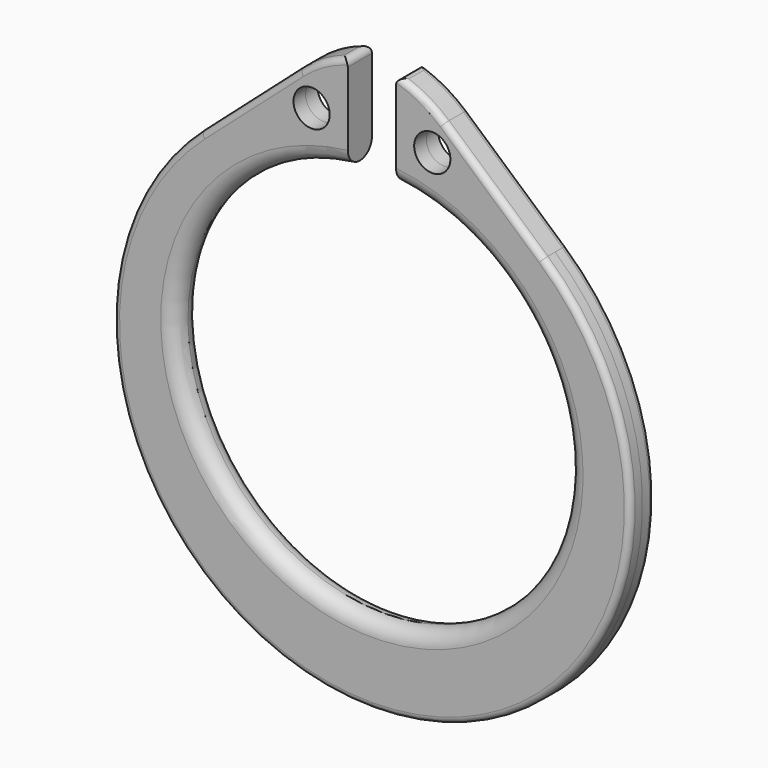
from build123d import *

# Parameters (mm, degrees)
F0_R     = 1.5
F1_DEPTH = 1.25
F2_R     = 1.24999
F3_R     = 0.5


# Not quite as in the source:
# - a fillet or chamfer is up to 0.001 mm smaller than in the source, because OpenCascade refuses the exact size


with BuildPart() as f1:
    # F0 (on Front) → F1 (new body, symmetric)
    with BuildSketch(Plane.XZ):
        with BuildLine():
            ThreePointArc((2, 16.1264534229), (0, -16.25), (-2, 16.1264534229))
            Line((-2, 16.1264534229), (-2, 24.1264534229))
            ThreePointArc((-2, 24.1264534229), (-4.1221023219, 23.2646436342), (-5.9979579511, 21.9504138084))
            Line((-5.9979579511, 21.9504138084), (-14.1837464065, 14.7155008072))
            ThreePointArc((-14.1837464065, 14.7155008072), (-20.0302422156, -8.9154770598), (0, -22.75))
            ThreePointArc((0, -22.75), (20.0302422156, -8.9154770598), (14.1837464065, 14.7155008072))
            Line((14.1837464065, 14.7155008072), (5.9979579511, 21.9504138084))
            ThreePointArc((5.9979579511, 21.9504138084), (4.1221023219, 23.2646436342), (2, 24.1264534229))
            Line((2, 24.1264534229), (2, 16.1264534229))
        make_face()
        with Locations((-5, 19.4933966718)):
            Circle(F0_R, mode=Mode.SUBTRACT)
        with Locations((5, 19.4933966718)):
            Circle(F0_R, mode=Mode.SUBTRACT)
    extrude(amount=F1_DEPTH, both=True)

    # F2 (radius 1.25 in the source; OpenCascade refuses exactly that, so slightly less here)
    f2_edges = [f1.edges().sort_by_distance(p)[0] for p in [
        (0, -1.25, -16.25),
        (0, 1.25, -16.25),
    ]]
    fillet(f2_edges, radius=F2_R)

    # F3
    f3_edges = [f1.edges().sort_by_distance(p)[0] for p in [
        (-20.030242, -1.25, -8.915477),
        (20.030242, -1.25, -8.915477),
        (-20.030242, 1.25, -8.915477),
        (20.030242, 1.25, -8.915477),
        (10.090852, 1.25, 18.332957),
        (10.090852, -1.25, 18.332957),
        (4.122102, -1.25, 23.264644),
        (4.122102, 1.25, 23.264644),
        (2, 0.625, 24.126453),
        (2, -0.625, 24.126453),
        (-10.090852, -1.25, 18.332957),
        (-10.090852, 1.25, 18.332957),
        (-4.122102, -1.25, 23.264644),
        (-4.122102, 1.25, 23.264644),
        (-2, 0.625, 24.126453),
        (-2, -0.625, 24.126453),
    ]]
    fillet(f3_edges, radius=F3_R)


solid = f1.part
